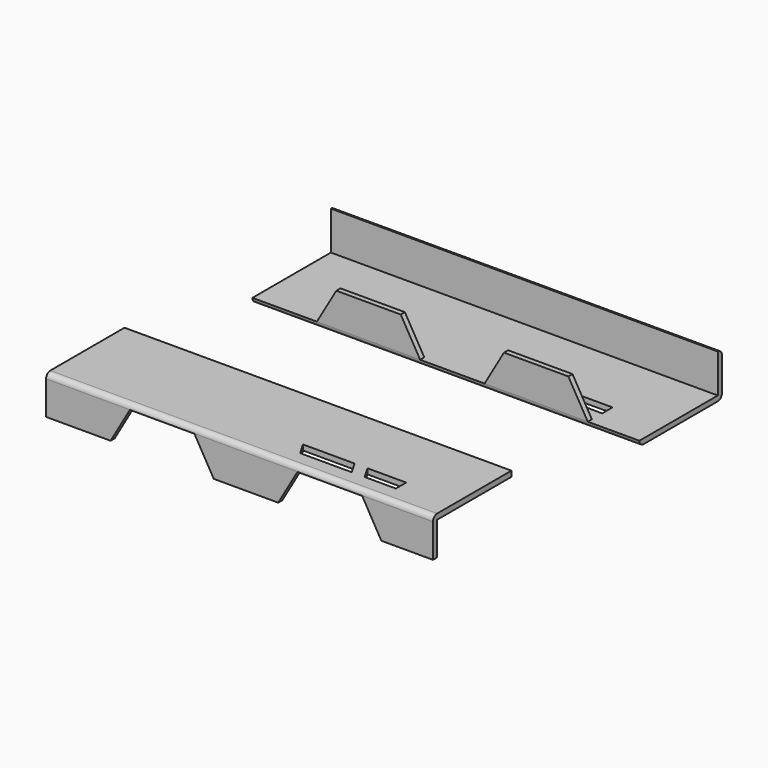
from build123d import *

# Parameters (mm, degrees)
F1_DEPTH  = 2
F4_DEPTH  = 2
F7_DEPTH  = 38
F10_DEPTH = 38
F11_W     = 150
F11_H     = 2
F12_DEPTH = 15
F13_W     = 2
F13_H     = 36
F14_DEPTH = 13
F16_DEPTH = 25
F18_DEPTH = 25
F19_R     = 1.99999
F19_2_R   = 1.99999
F20_R     = 1.99999


# Not quite as in the source:
# - a fillet or chamfer is up to 0.001 mm smaller than in the source, because OpenCascade refuses the exact size


with BuildPart() as f1:
    # F0 (on Front) → F1 (new body)
    with BuildSketch(Plane.XZ):
        Polygon((-76.9333613626, -12.8761603036), (-101.9333613626, -12.8761603036), (-101.9333613626, -14.8761603036), (48.0666386374, -14.8761603036), (48.0666386374, -12.8761603036), (28.0555316385, -12.8761603036), (20.549978139, 0.1238396964), (-4.438914862, 0.1238396964), (-11.9444683615, -12.8761603036), (-36.9333613626, -12.8761603036), (-44.438914862, 0.1238396964), (-69.4278078631, 0.1238396964), align=None)
    extrude(amount=F1_DEPTH)

    # F6 (on offset) → F7 (join, through all)
    with BuildSketch(Plane.XZ.offset(-38)):
        Polygon((-36.9333613626, -12.8761603036), (-76.9333613626, -12.8761603036), (-101.9333613626, -12.8761603036), (-101.9333613626, -14.8761603036), (48.0666386374, -14.8761603036), (48.0666386374, -12.8761603036), (28.0555316385, -12.8761603036), (-11.9444683615, -12.8761603036), align=None)
    extrude(amount=F7_DEPTH)

    # F11 (on face) → F12 (join)
    with BuildSketch(Plane.XY.offset(-12.8761603036)):
        with Locations((-26.9333613626, 37)):
            Rectangle(F11_W, F11_H)
    extrude(amount=F12_DEPTH)

    # F17 (on face) → F18 (cut)
    with BuildSketch(Plane(origin=(0, 0, -14.8761603036), x_dir=(1, 0, 0), z_dir=(0, 0, -1))):
        Polygon((-11.9333613626, -10), (8.0666386374, -10), (10.9533899834, -5), (-9.0466100166, -5), align=None)
        Polygon((13.0666386374, -10), (28.0666386374, -10), (28.0666386374, -5), (15.9533899834, -5), align=None)
    extrude(amount=-F18_DEPTH, mode=Mode.SUBTRACT)

    # F19 (radius 2 in the source; OpenCascade refuses exactly that, so slightly less here)
    f19_edges = [f1.edges().sort_by_distance(p)[0] for p in [
        (-26.933361, 38, -14.87616),
        (-26.933361, 38, 2.12384),
    ]]
    fillet(f19_edges, radius=F19_R)

    # F20 (radius 2 in the source; OpenCascade refuses exactly that, so slightly less here)
    f20_edges = [f1.edges().sort_by_distance(p)[0] for p in [
        (-26.933361, -2, -14.87616),
    ]]
    fillet(f20_edges, radius=F20_R)


with BuildPart() as f4:
    # F3 (on offset) → F4 (new body)
    with BuildSketch(Plane.XZ.offset(100)):
        Polygon((-101.9333613626, 0.1238396964), (-101.9333613626, -12.8761603036), (-76.9333613626, -12.8761603036), (-69.4278078631, 0.1238396964), (-44.438914862, 0.1238396964), (-36.9333613626, -12.8761603036), (-11.9444683615, -12.8761603036), (-4.438914862, 0.1238396964), (20.549978139, 0.1238396964), (28.0555316385, -12.8761603036), (48.0666386374, -12.8761603036), (48.0666386374, 0.1238396964), (48.0666386374, 2.1238396964), (-101.9333613626, 2.1238396964), align=None)
    extrude(amount=F4_DEPTH)

    # F9 (on offset) → F10 (join)
    with BuildSketch(Plane.XZ.offset(64)):
        Polygon((48.0666386374, 2.1238396964), (-101.9333613626, 2.1238396964), (-101.9333613626, 0.1238396964), (-69.4432945528, 0.097015963), (-44.4114965352, 0.0763497612), (-4.4853643477, 0.0433868273), (20.6083887933, 0.0226694755), (48.0666386374, 0), align=None)
    extrude(amount=F10_DEPTH)

    # F13 (on face) → F14 (join)
    with BuildSketch(Plane(origin=(3.27628e-05, 0, 0.0396836925), x_dir=(0.9999996592, 0, -0.0008255977), z_dir=(-0.0008255977, 0, -0.9999996592))):
        with Locations((-100.9334288649, 82)):
            Rectangle(F13_W, F13_H)
    extrude(amount=F14_DEPTH)

    # F15 (on face) → F16 (cut)
    with BuildSketch(Plane.XY.offset(2.1238396964)):
        Polygon((10.9533899834, -95), (8.0666386374, -90), (-11.9333613626, -90), (-9.0466100166, -95), align=None)
        Polygon((28.0666386374, -95), (28.0666386374, -90), (13.0666386374, -90), (15.9533899834, -95), align=None)
    extrude(amount=-F16_DEPTH, mode=Mode.SUBTRACT)

    # F19#2 (radius 2 in the source; OpenCascade refuses exactly that, so slightly less here)
    f19_2_edges = [f4.edges().sort_by_distance(p)[0] for p in [
        (-26.933361, -102, 2.12384),
    ]]
    fillet(f19_2_edges, radius=F19_2_R)


solid = Compound([f1.part, f4.part])
